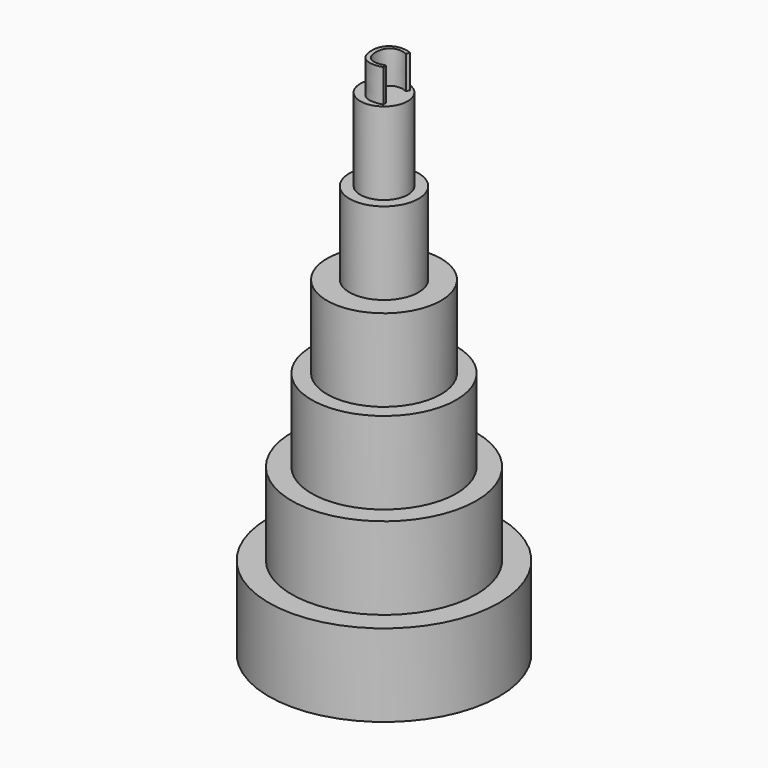
from build123d import *

# Parameters (mm, degrees)
F0_R          = 17.7473728483
F1_DEPTH      = 12.7
F2_R          = 14.2238366896
F3_DEPTH      = 25.4
F4_R          = 11.1559536629
F5_DEPTH      = 38.1
F6_R          = 8.7886851069
F7_DEPTH      = 50.8
F8_R          = 5.3263507997
F9_DEPTH      = 63.5
F10_R         = 3.6612500332
F11_DEPTH     = 76.2
F12_TEXT_SIZE = 7.4135078143
F13_DEPTH     = 81.28


# Not quite as in the source:
# - Text() gives the source's letters only with a copy of the font that has no kerning and outlines rounded to 1/6400 em; it was checked with that copy


with BuildPart() as f1:
    # F0 (on Top) → F1 (new body)
    with BuildSketch(Plane.XY):
        Circle(F0_R)
    extrude(amount=F1_DEPTH)

    # F2 (on Top) → F3 (join)
    with BuildSketch(Plane.XY):
        Circle(F2_R)
    extrude(amount=F3_DEPTH)

    # F4 (on Top) → F5 (join)
    with BuildSketch(Plane.XY):
        Circle(F4_R)
    extrude(amount=F5_DEPTH)

    # F6 (on Top) → F7 (join)
    with BuildSketch(Plane.XY):
        Circle(F6_R)
    extrude(amount=F7_DEPTH)

    # F8 (on Top) → F9 (join)
    with BuildSketch(Plane.XY):
        Circle(F8_R)
    extrude(amount=F9_DEPTH)

    # F10 (on Top) → F11 (join)
    with BuildSketch(Plane.XY):
        Circle(F10_R)
    extrude(amount=F11_DEPTH)

    # F12 (on Top) → F13 (join)
    with BuildSketch(Plane.XY):
        with Locations((-2.3455267074, -2.6502651162)):
            Text('C', F12_TEXT_SIZE, font='Open Sans', text_align=(TextAlign.LEFT, TextAlign.BOTTOM))
    extrude(amount=F13_DEPTH)


solid = f1.part
